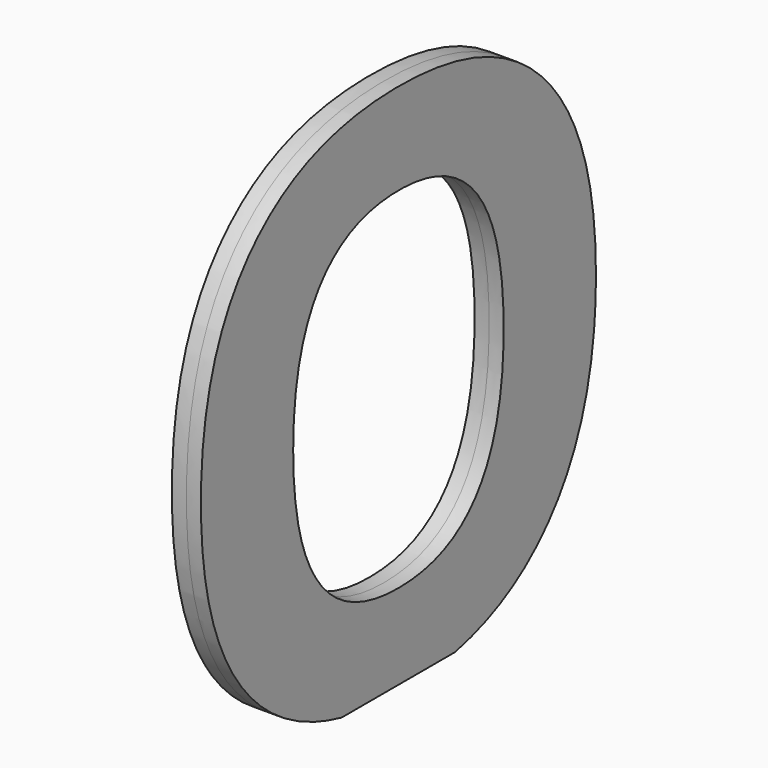
from build123d import *

# Parameters (mm, degrees)
F0_TEXT_SIZE = 635
F1_DEPTH     = 12.7
F2_W         = 456.5707343619
F2_H         = 78.4809016315
F3_DEPTH     = 25.4010001


# Not quite as in the source:
# - Text() gives the source's letters only with a copy of the font that has no kerning and outlines rounded to 1/6400 em; it was checked with that copy


with BuildPart() as f1:
    # F0 (on Right) → F1 (new body, symmetric)
    with BuildSketch(Plane.YZ):
        with Locations((-164.9192172091, -269.0176046761)):
            Text('O', F0_TEXT_SIZE, font='Open Sans', font_style=FontStyle.BOLD, text_align=(TextAlign.LEFT, TextAlign.BOTTOM))
    extrude(amount=F1_DEPTH, both=True)

    # F2 (on face) → F3 (cut, through all)
    with BuildSketch(Plane.YZ.offset(12.7)):
        with Locations((63.3661499719, -308.2580554918)):
            Rectangle(F2_W, F2_H)
    extrude(amount=-F3_DEPTH, mode=Mode.SUBTRACT)


solid = f1.part
